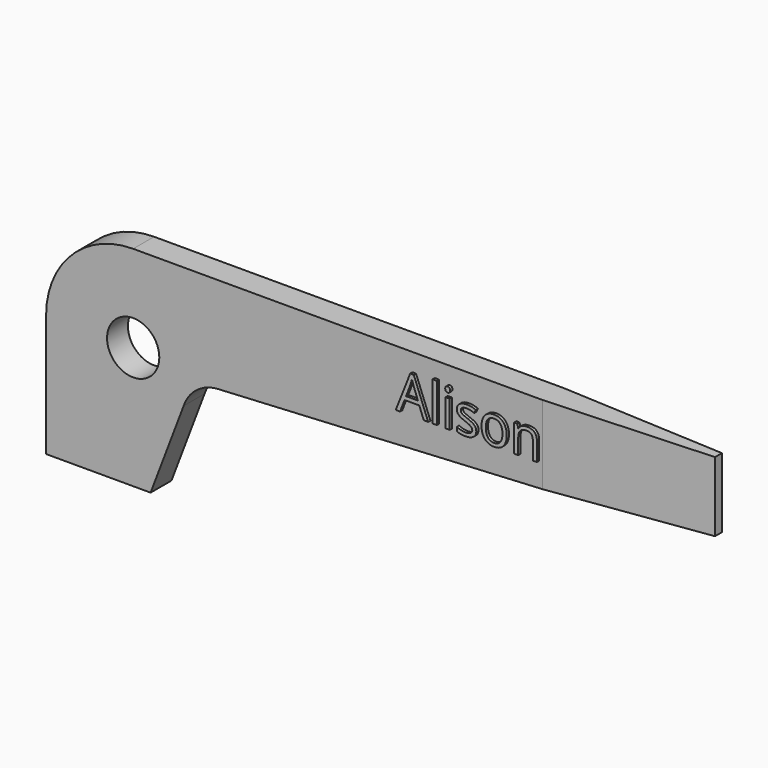
from build123d import *

# Parameters (mm, degrees)
F1_DEPTH     = 2.38125
F2_R         = 2.38125
F3_DEPTH     = 25.4
F5_DEPTH     = 25.4
F6_TEXT_SIZE = 4.6744683964
F7_DEPTH     = 0.254


# Not quite as in the source:
# - Text() gives the source's letters only with a copy of the font that has no kerning and outlines rounded to 1/6400 em; it was checked with that copy


with BuildPart() as f1:
    # F0 (on Front) → F1 (new body)
    with BuildSketch(Plane.XZ):
        with BuildLine():
            Line((60.325, 19.05), (7.9375, 19.05))
            ThreePointArc((7.9375, 19.05), (2.3248399243, 16.7251600757), (0, 11.1125))
            Line((0, 11.1125), (0, 0))
            Line((0, 0), (9.525, 0))
            Line((9.525, 0), (12.5373871997, 7.9435762018))
            ThreePointArc((12.5373871997, 7.9435762018), (13.7368903476, 9.6077253312), (15.6631963617, 10.3130942181))
            Line((15.6631963617, 10.3130942181), (60.325, 12.7))
            Line((60.325, 12.7), (60.325, 19.05))
        make_face()
    extrude(amount=F1_DEPTH)

    # F2 (on face) → F3 (cut)
    with BuildSketch(Plane.XZ.offset(2.38125)):
        with Locations((7.9375, 11.1125)):
            Circle(F2_R)
    extrude(amount=-F3_DEPTH, mode=Mode.SUBTRACT)

    # F4 (on face) → F5 (cut)
    with BuildSketch(Plane.XY.offset(19.05)):
        Polygon((60.325, 0), (45.24375, 0), (60.325, -0.79375), align=None)
        Polygon((60.325, -2.38125), (60.325, -1.5875), (45.24375, -2.38125), align=None)
    extrude(amount=-F5_DEPTH, mode=Mode.SUBTRACT)

    # F6 (on face) → F7 (join)
    with BuildSketch(Plane.XZ.offset(2.38125)):
        with Locations((32.071244136, 14.0699949116)):
            Text('Alison', F6_TEXT_SIZE, font='Open Sans', text_align=(TextAlign.LEFT, TextAlign.BOTTOM))
    extrude(amount=F7_DEPTH)


solid = f1.part
